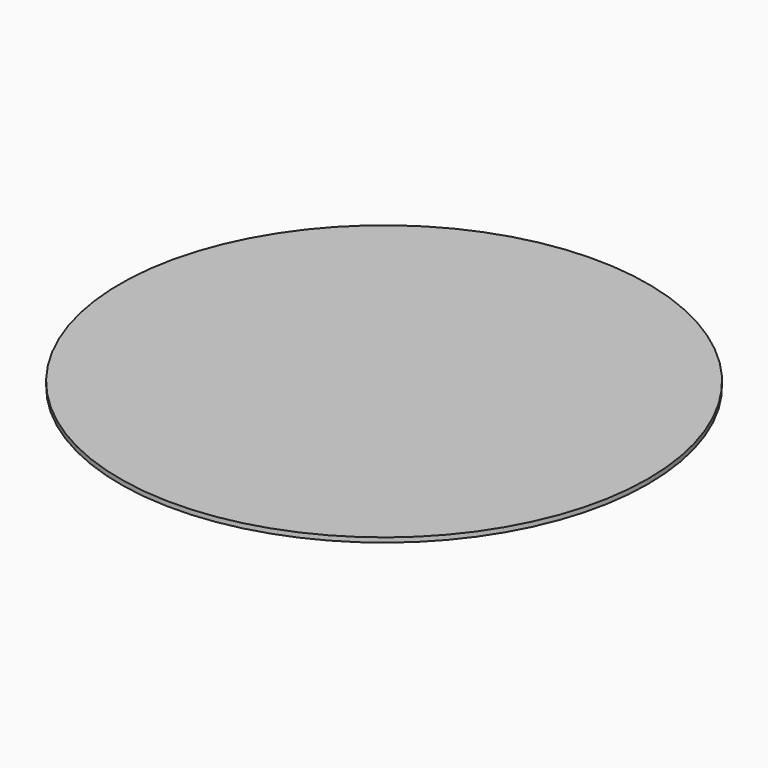
from build123d import *

# Parameters (mm, degrees)
F0_R = 152.4


# Not quite as in the source:
# - the program builds the solid bodies; features that only make, move or delete a surface that nothing else refers to are left out


with BuildPart() as f2:
    # F2: sweep along a path in F1
    with BuildLine(Plane.XZ) as f2_path:
        Line((0, 0), (0, 2.6722908951))
    # F0 (on Top) → F2 (sweep)
    with BuildSketch(Plane.XY):
        with Locations((0.2868945012, -3.5133e-06)):
            Circle(F0_R)
    sweep(path=f2_path.line)


solid = f2.part
